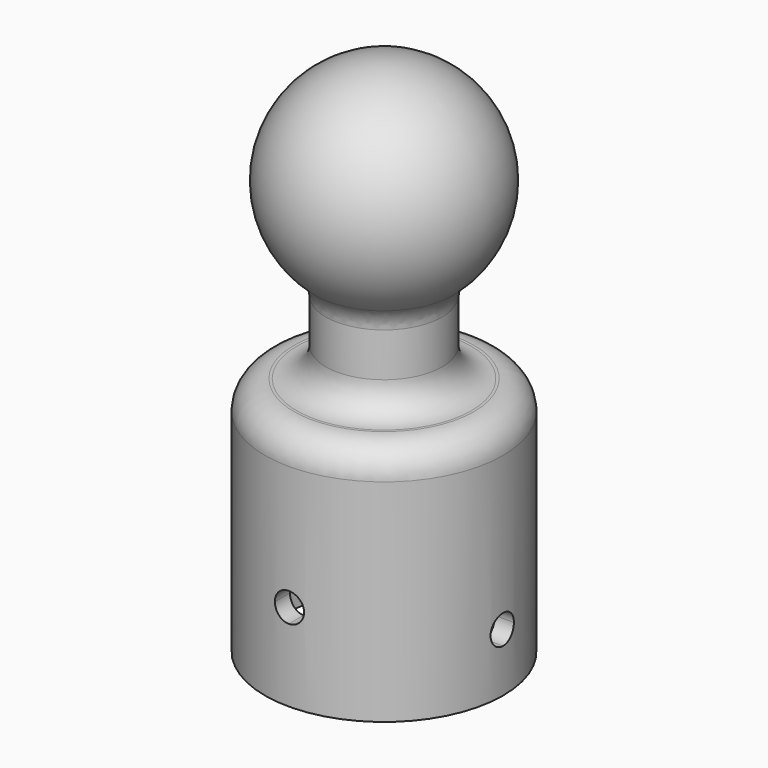
from build123d import *

# Parameters (mm, degrees)
F2_R      = 10
F2_R_2    = 5
F3_DEPTH  = 15
F6_R      = 5
F7_W      = 5
F7_H      = 5
F8_DEPTH  = 25
F9_W      = 5
F9_H      = 5
F10_DEPTH = 25
F11_R     = 2.499


# Not quite as in the source:
# - a fillet or chamfer is up to 0.001 mm smaller than in the source, because OpenCascade refuses the exact size


with BuildPart() as f1:
    # F0 (on Front) → F1 (revolve)
    with BuildSketch(Plane.XZ):
        with BuildLine():
            Line((17.25, 33.1), (17.25, 0))
            Line((17.25, 0), (20.45, 0))
            Line((20.45, 0), (20.45, 41.3))
            Line((20.45, 41.3), (0, 41.3))
            Line((0, 41.3), (0, 38.1))
            Line((0, 38.1), (12.25, 38.1))
            ThreePointArc((12.25, 38.1), (15.7855339059, 36.6355339059), (17.25, 33.1))
        make_face()
    revolve(axis=Axis((0, 0, 39.7), (0, 0, 1)))

    # F2 (on face) → F3 (join)
    with BuildSketch(Plane.XY.offset(41.3)):
        Circle(F2_R)
        Circle(F2_R_2, mode=Mode.SUBTRACT)
    extrude(amount=F3_DEPTH)

    # F4 (on Front) → F5 (revolve)
    with BuildSketch(Plane.XZ):
        with BuildLine():
            Line((0, 56.3), (10, 56.3))
            ThreePointArc((10, 56.3), (17.2249721603, 76.4916017074), (0, 89.2666295471))
            Line((0, 89.2666295471), (0, 81.2666295471))
            ThreePointArc((0, 81.2666295471), (10, 71.2666295471), (0, 61.2666295471))
            Line((0, 61.2666295471), (0, 56.3))
        make_face()
    revolve(axis=Axis((0, 0, 85.2666295471), (0, 0, -1)))

    # F6
    f6_edges = [f1.edges().sort_by_distance(p)[0] for p in [
        (-10, 0, 56.3),
        (-20.45, 0, 41.3),
        (-10, 0, 41.3),
    ]]
    fillet(f6_edges, radius=F6_R)

    # F7 (on Front) → F8 (cut, symmetric)
    with BuildSketch(Plane.XZ):
        with Locations((0, 15)):
            Rectangle(F7_W, F7_H)
    extrude(amount=F8_DEPTH, both=True, mode=Mode.SUBTRACT)

    # F9 (on Right) → F10 (cut, symmetric)
    with BuildSketch(Plane.YZ):
        with Locations((0, 10)):
            Rectangle(F9_W, F9_H)
    extrude(amount=F10_DEPTH, both=True, mode=Mode.SUBTRACT)

    # F11 (radius 2.5 in the source; OpenCascade refuses exactly that, so slightly less here)
    f11_edges = [f1.edges().sort_by_distance(p)[0] for p in [
        (18.682246, -2.5, 12.5),
        (-18.682246, -2.5, 12.5),
        (18.682246, -2.5, 7.5),
        (-18.682246, -2.5, 7.5),
        (18.682246, 2.5, 7.5),
        (-18.682246, 2.5, 7.5),
        (18.682246, 2.5, 12.5),
        (-18.682246, 2.5, 12.5),
        (-2.5, 18.682246, 17.5),
        (-2.5, -18.682246, 17.5),
        (-2.5, 18.682246, 12.5),
        (-2.5, -18.682246, 12.5),
        (2.5, 18.682246, 12.5),
        (2.5, -18.682246, 12.5),
        (2.5, 18.682246, 17.5),
        (2.5, -18.682246, 17.5),
    ]]
    fillet(f11_edges, radius=F11_R)


solid = f1.part
